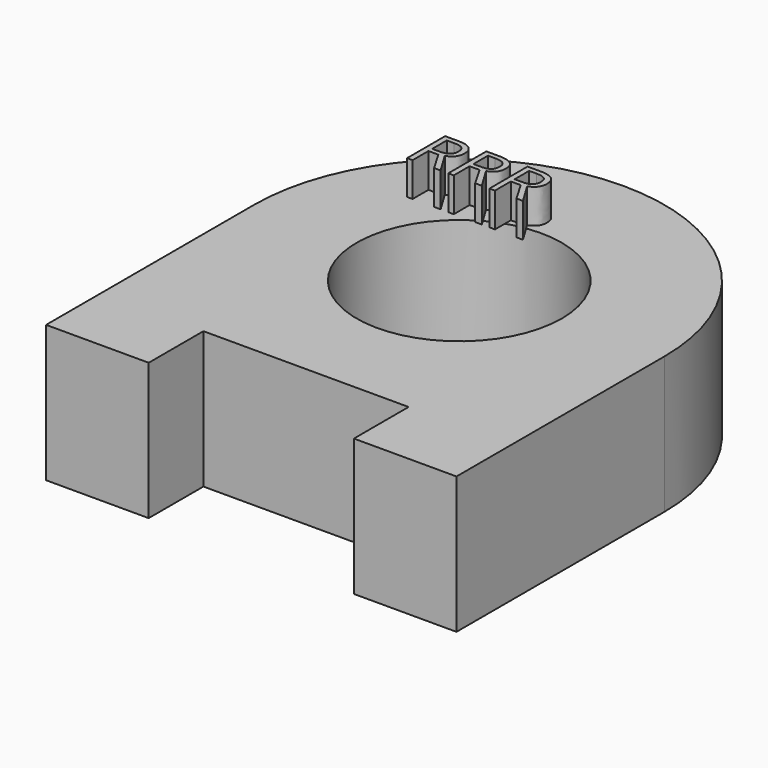
from build123d import *

# Parameters (mm, degrees)
F0_R         = 15
F1_DEPTH     = 20
F2_TEXT_SIZE = 9.7401634169
F3_DEPTH     = 5


# Not quite as in the source:
# - Text() gives the source's letters only with a copy of the font that has no kerning and outlines rounded to 1/6400 em; it was checked with that copy


with BuildPart() as f1:
    # F0 (on Top) → F1 (new body)
    with BuildSketch(Plane.XY):
        with BuildLine():
            Line((30, -38), (30, 0))
            ThreePointArc((30, 0), (0, 30), (-30, 0))
            Line((-30, 0), (-30, -38))
            Line((-30, -38), (-15, -38))
            Line((-15, -38), (-15, -28))
            Line((-15, -28), (15, -28))
            Line((15, -28), (15, -38))
            Line((15, -38), (30, -38))
        make_face()
        Circle(F0_R, mode=Mode.SUBTRACT)
    extrude(amount=F1_DEPTH)

    # F2 (on face) → F3 (join)
    with BuildSketch(Plane.XY.offset(20)):
        with Locations((-18.5276170996, 12.4349584803)):
            Text('RRR', F2_TEXT_SIZE, font='Open Sans', text_align=(TextAlign.LEFT, TextAlign.BOTTOM))
    extrude(amount=F3_DEPTH)


solid = f1.part
